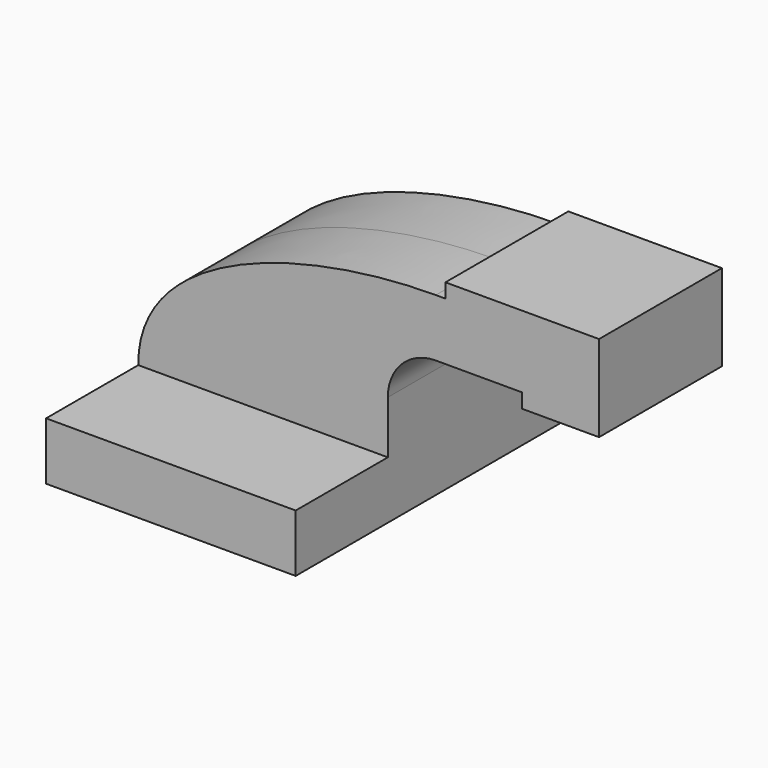
from build123d import *

# Parameters (mm, degrees)
F0_W     = 82.55
F0_H     = 19.05
F1_DEPTH = 63.5
F2_DEPTH = 25.4
F0_W_2   = 25.4
F3_DEPTH = 25.4
F4_DEPTH = 25.4
F0_H_2   = 4.7498
F5_DEPTH = 25.4


with BuildPart() as f1:
    # F0 (on Front) → F1 (new body, symmetric)
    with BuildSketch(Plane.XZ):
        Rectangle(F0_W, F0_H)
    extrude(amount=F1_DEPTH, both=True)

    # F0 (on Front) → F2 (join, symmetric)
    with BuildSketch(Plane.XZ):
        with BuildLine():
            Line((-41.275, 9.525), (41.275, 9.525))
            Line((41.275, 9.525), (41.275, 27.0002))
            ThreePointArc((41.275, 27.0002), (45.9246798487, 38.2255201513), (57.15, 42.8752))
            Line((57.15, 42.8752), (60.325, 42.8752))
            Line((60.325, 42.8752), (60.325, 61.9252))
            Line((60.325, 61.9252), (57.15, 61.9252))
            add(Edge.make_bspline(
                [(-41.275, 9.525), (-41.5499731898, 46.1455024779), (14.5141012144, 61.9252), (57.15, 61.9252)],
                knots=[0, 0, 0, 0, 111.5045361635, 111.5045361635, 111.5045361635, 111.5045361635], degree=3))
        make_face()
    extrude(amount=F2_DEPTH, both=True)

    # F0 (on Front) → F3 (join, symmetric)
    with BuildSketch(Plane.XZ):
        with Locations((73.025, 52.4002)):
            Rectangle(F0_W_2, F0_H)
    extrude(amount=F3_DEPTH, both=True)

    # F0 (on Front) → F4 (join, symmetric)
    with BuildSketch(Plane.XZ):
        Polygon((85.725, 66.675), (85.725, 61.9252), (85.725, 42.8752), (85.725, 38.1), (111.125, 38.1), (111.125, 66.675), align=None)
    extrude(amount=F4_DEPTH, both=True)

    # F0 (on Front) → F5 (join, symmetric)
    with BuildSketch(Plane.XZ):
        with Locations((73.025, 64.3001)):
            Rectangle(F0_W_2, F0_H_2)
    extrude(amount=F5_DEPTH, both=True)


solid = f1.part
